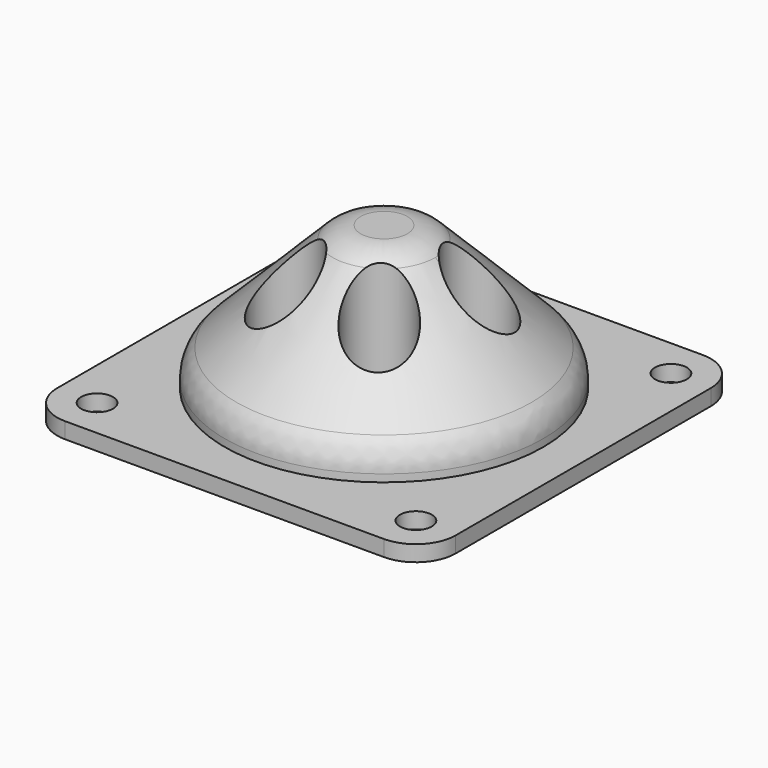
from build123d import *

# Parameters (mm, degrees)
F0_R     = 20
F0_R_2   = 4
F1_DEPTH = 20
F0_W     = 50
F0_H     = 50
F3_DEPTH = 2
F4_R     = 5
F5_D     = 4
F7_SIZE2 = 6
F7_SIZE  = 1
F8_R     = 5


# Not quite as in the source:
# - a fillet or chamfer that OpenCascade refuses, or shapes differently, is made with other operations: its cross-section is extruded or revolved along the edge and cut away or added


with BuildPart() as f1:
    # F0 (on Top) → F1 (new body)
    with BuildSketch(Plane.XY):
        Circle(F0_R)
        with Locations((-5.8778525229, -8.0901699437)):
            Circle(F0_R_2, mode=Mode.SUBTRACT)
        with Locations((5.8778525229, -8.0901699437)):
            Circle(F0_R_2, mode=Mode.SUBTRACT)
        with Locations((-9.510565163, 3.0901699437)):
            Circle(F0_R_2, mode=Mode.SUBTRACT)
        with Locations((9.510565163, 3.0901699437)):
            Circle(F0_R_2, mode=Mode.SUBTRACT)
        with Locations((0, 10)):
            Circle(F0_R_2, mode=Mode.SUBTRACT)
    extrude(amount=F1_DEPTH)

    # F2: chamfer of 15 on 1 edges, made by hand

    # F2_s1 → F2_t2 (revolve, cut)
    with BuildSketch(Plane.XZ):
        Polygon((20, 5), (5, 20), (20, 20), align=None)
    revolve(axis=Axis((0, 0, 20), (0, 0, 1)), mode=Mode.SUBTRACT)

    # F0 (on Top) → F3 (join)
    with BuildSketch(Plane.XY):
        Rectangle(F0_W, F0_H)
        Circle(F0_R, mode=Mode.SUBTRACT)
    extrude(amount=F3_DEPTH)

    # F4
    f4_edges = [f1.edges().sort_by_distance(p)[0] for p in [
        (-25, 25, 1),
        (25, 25, 1),
        (25, -25, 1),
        (-25, -25, 1),
    ]]
    fillet(f4_edges, radius=F4_R)

    # F5 (through all)
    with Locations(Plane(origin=(0, 0, 0), x_dir=(1, 0, 0), z_dir=(0, 0, -1))):
        with Locations((-20, -20), (20, -20), (20, 20), (-20, 20)):
            Hole(F5_D / 2)

    # F6: fillet of radius 5 on 1 edges, made by hand

    # F6_s1 → F6_t2 (revolve, cut)
    with BuildSketch(Plane.XZ):
        with BuildLine():
            ThreePointArc((6.4644660941, 18.5355339059), (4.84234935, 19.6193976626), (2.9289321881, 20))
            Line((2.9289321881, 20), (5, 20))
            Line((5, 20), (6.4644660941, 18.5355339059))
        make_face()
    revolve(axis=Axis((0, 0, 20), (0, 0, 1)), mode=Mode.SUBTRACT)

    # F7
    f7_edges = [f1.edges().sort_by_distance(p)[0] for p in [
        (5.510565, 3.09017, 0),
        (-4, 10, 0),
        (-13.510565, 3.09017, 0),
        (-9.877853, -8.09017, 0),
        (1.877853, -8.09017, 0),
    ]]
    f7_side = f1.faces().sort_by_distance((0, 0, 0))[0]
    chamfer(f7_edges, length=F7_SIZE, length2=F7_SIZE2, reference=f7_side)

    # F8
    f8_edges = [f1.edges().sort_by_distance(p)[0] for p in [
        (-20, 0, 5),
    ]]
    fillet(f8_edges, radius=F8_R)


solid = f1.part
